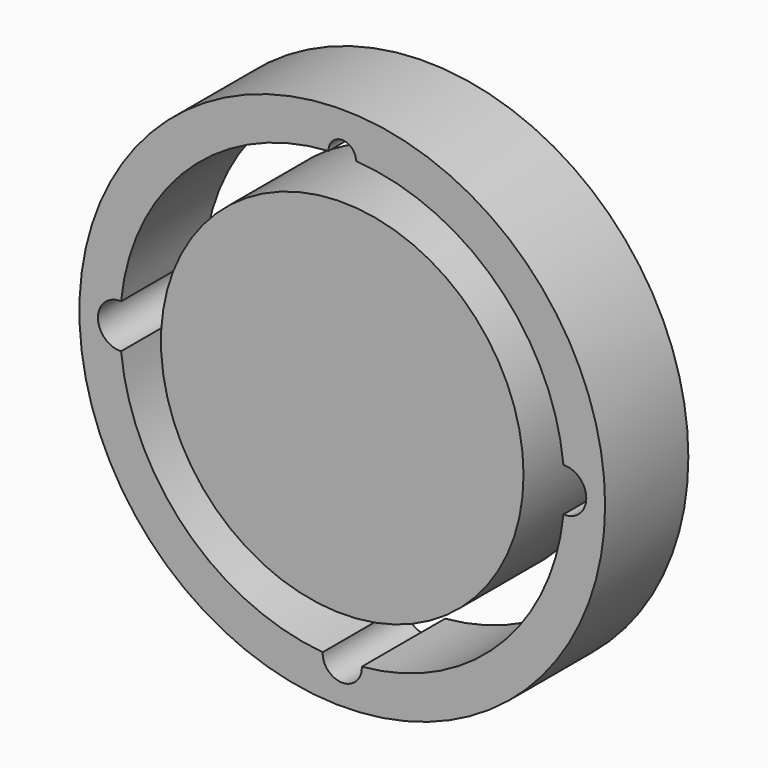
from build123d import *

# Parameters (mm, degrees)
F0_R     = 32.0777446032
F1_DEPTH = 12.7
F0_R_2   = 22.1233486921


# Not quite as in the source:
# - a feature of the source that left no trace in its solid (it failed there, or was rolled back) is left out
# - a feature names something its author has since deleted; it is built from what else it names


with BuildPart() as f1:
    # F0 (on Front) → F1 (new body)
    with BuildSketch(Plane.XZ):
        Circle(F0_R)
        with BuildLine():
            ThreePointArc((1.6706113004, 27.0691254094), (18.8235281215, 19.5244278176), (26.9899975467, 2.658669775))
            ThreePointArc((26.9899975467, 2.658669775), (28.9560938487, 1.9278632057), (29.7825055927, 0))
            ThreePointArc((29.7825055927, 0), (28.9560938487, -1.9278632057), (26.9899975467, -2.658669775))
            ThreePointArc((26.9899975467, -2.658669775), (19.0808918692, -19.2729877814), (2.3881836562, -27.0152747787))
            ThreePointArc((2.3881836562, -27.0152747787), (2.3899256032, -27.0679388604), (2.3905063462, -27.1206285426))
            ThreePointArc((2.3905063462, -27.1206285426), (-0.0526896822, -29.5105541458), (-2.3881836562, -27.0152747787))
            ThreePointArc((-2.3881836562, -27.0152747787), (-19.0715734338, -19.2822088804), (-26.9874146305, -2.684761462))
            ThreePointArc((-26.9874146305, -2.684761462), (-29.8086929121, 0), (-26.9874146305, 2.684761462))
            ThreePointArc((-26.9874146305, 2.684761462), (-18.8140881746, 19.5335244824), (-1.6706113004, 27.0691254094))
            ThreePointArc((-1.6706113004, 27.0691254094), (-0.0257546243, 28.7918351095), (1.6714050047, 27.1206285426))
            ThreePointArc((1.6714050047, 27.1206285426), (1.6712065668, 27.0948739183), (1.6706113004, 27.0691254094))
        make_face(mode=Mode.SUBTRACT)
    extrude(amount=F1_DEPTH)


with BuildPart() as f1b:
    # F0 (on Front) → F1, piece 2 (new body)
    with BuildSketch(Plane.XZ):
        Circle(F0_R_2)
    extrude(amount=F1_DEPTH)


solid = Compound([f1.part, f1b.part])
